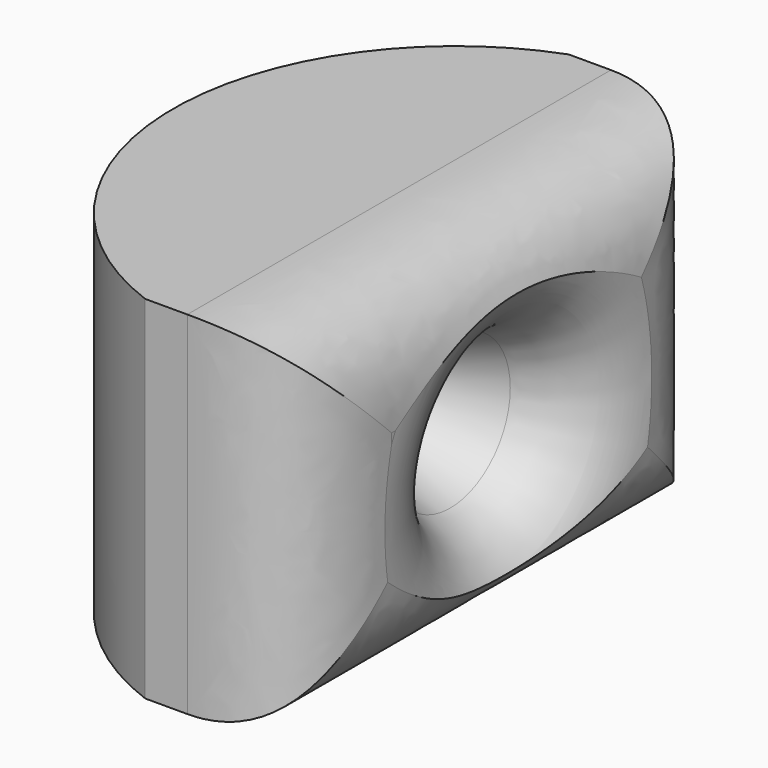
from build123d import *

# Parameters (mm, degrees)
F1_DEPTH    = 47.244
F2_R        = 13.7417577373
F4_T1_DEPTH = 123.444
F4_T3_DEPTH = 147.3045786738


# Not quite as in the source:
# - a fillet or chamfer that OpenCascade refuses, or shapes differently, is made with other operations: its cross-section is extruded or revolved along the edge and cut away or added
# - an extrude whose draft closes it to a point is written as a loft to that point


with BuildPart() as f1:
    # F0 (on Top) → F1 (new body)
    with BuildSketch(Plane.XY):
        with BuildLine():
            Line((-38.2979549468, 31.997974962), (-59.2006028914, 31.997974962))
            ThreePointArc((-59.2006028914, 31.997974962), (-83.8900545196, -3.5543143749), (-59.2006028914, -39.1066037118))
            Line((-59.2006028914, -39.1066037118), (-38.2979549468, -39.1066037118))
            Line((-38.2979549468, -39.1066037118), (-38.2979549468, 31.997974962))
        make_face()
    extrude(amount=F1_DEPTH)

    # F2 (on face) → F3 section 0
    with BuildSketch(Plane.YZ.offset(-38.2979549468), mode=Mode.PRIVATE) as f3_s0:
        with Locations((-1.4992692741, 20.8444874734)):
            Circle(F2_R)
    loft([f3_s0.sketch, Vertex(-76.0531240335, -1.4992692741, 20.8444874734)], ruled=True, mode=Mode.SUBTRACT)

    # F4: fillet of radius 15.24 on 5 edges, made by hand

    # F4_s2 → F4_t1 (cut)
    with BuildSketch(Plane.XY.offset(-38.1)):
        with BuildLine():
            add(Edge.make_bspline(
                [(-53.5379549468, -39.1066037118), (-38.2979549468, -39.1066037118), (-38.2979549468, -23.8666037118)],
                knots=[0, 0, 0, 1, 1, 1], degree=2, weights=[1, 1, 1]))
            Line((-38.2979549468, -23.8666037118), (-38.2979549468, -39.1066037118))
            Line((-38.2979549468, -39.1066037118), (-53.5379549468, -39.1066037118))
        make_face()
        with BuildLine():
            add(Edge.make_bspline(
                [(-53.5379549468, 31.997974962), (-38.2979549468, 31.997974962), (-38.2979549468, 16.757974962)],
                knots=[0, 0, 0, 1, 1, 1], degree=2, weights=[1, 1, 1]))
            Line((-38.2979549468, 16.757974962), (-38.2979549468, 31.997974962))
            Line((-38.2979549468, 31.997974962), (-53.5379549468, 31.997974962))
        make_face()
    extrude(amount=F4_T1_DEPTH, mode=Mode.SUBTRACT)

    # F4_s4 → F4_t3 (cut)
    with BuildSketch(Plane.XZ.offset(-70.097974962)):
        with BuildLine():
            add(Edge.make_bspline(
                [(-53.5379549468, 0), (-38.2979549468, 0), (-38.2979549468, 15.24)],
                knots=[0, 0, 0, 1, 1, 1], degree=2, weights=[1, 1, 1]))
            Line((-38.2979549468, 15.24), (-38.2979549468, 0))
            Line((-38.2979549468, 0), (-53.5379549468, 0))
        make_face()
        with BuildLine():
            add(Edge.make_bspline(
                [(-53.5379549468, 47.244), (-38.2979549468, 47.244), (-38.2979549468, 32.004)],
                knots=[0, 0, 0, 1, 1, 1], degree=2, weights=[1, 1, 1]))
            Line((-38.2979549468, 32.004), (-38.2979549468, 47.244))
            Line((-38.2979549468, 47.244), (-53.5379549468, 47.244))
        make_face()
    extrude(amount=F4_T3_DEPTH, mode=Mode.SUBTRACT)

    # F4_s5 → F4_t6 (revolve, cut)
    with BuildSketch(Plane.XY.offset(20.8444874734)):
        with BuildLine():
            add(Edge.make_bspline(
                [(-38.2979549468, 22.9136513455), (-38.2979549468, 12.2424884632), (-48.3255679625, 8.5927358047)],
                knots=[0, 0, 0, 1, 1, 1], degree=2, weights=[1, 1, 1]))
            Line((-48.3255679625, 8.5927358047), (-38.2979549468, 12.2424884632))
            Line((-38.2979549468, 12.2424884632), (-38.2979549468, 22.9136513455))
        make_face()
    revolve(axis=Axis((-38.2979549468, -1.4992692741, 20.8444874734), (1, 0, 0)), mode=Mode.SUBTRACT)


solid = f1.part
